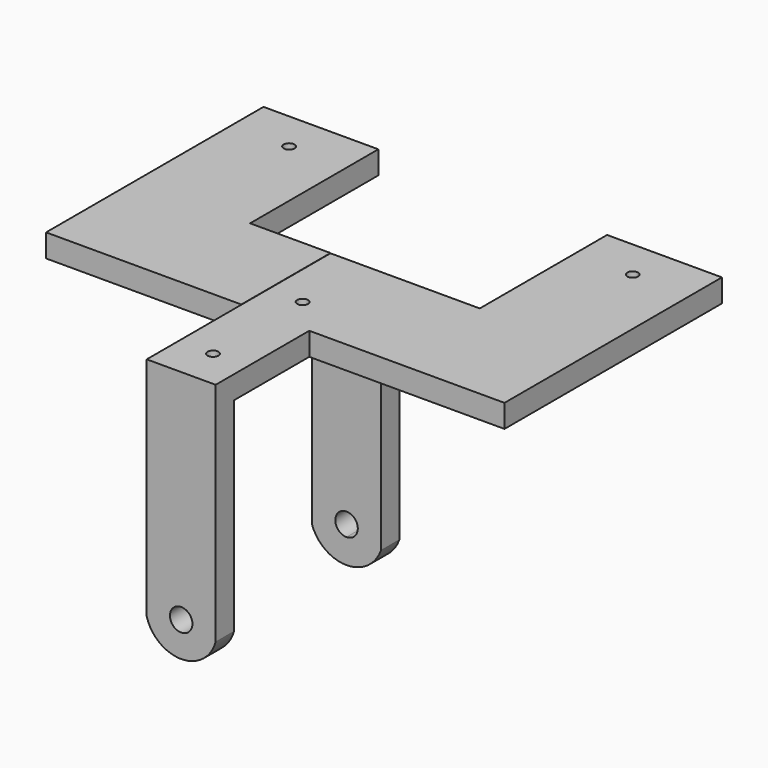
from build123d import *

# Parameters (mm, degrees)
F1_DEPTH  = 3.175
F2_DEPTH  = 3.175
F4_DEPTH  = 25.4
F5_DEPTH  = 25.4
F6_W      = 19.05
F6_H      = 63.5
F7_DEPTH  = 6.35
F9_DEPTH  = 6.35
F10_DEPTH = 2540
F11_R     = 1.5
F12_DEPTH = 25.4
F13_W     = 75.1403903484
F13_H     = 6.35
F14_DEPTH = 53.975
F15_R     = 1.5
F16_DEPTH = 25
F17_W     = 75.1403903484
F17_H     = 6.35
F18_DEPTH = 53.975
F19_R     = 1.5
F20_DEPTH = 25
F22_DEPTH = 22.225
F23_W     = 44.3243741632
F23_H     = 6.35
F24_DEPTH = 22.225


# Not quite as in the source:
# - a length typed as a fraction of an inch, garbled in the dataset ("3 / 203.2 mm" for 3/8 in), is restored


with BuildPart() as f1:
    # F0 (on Front) → F1 (new body)
    with BuildSketch(Plane.XZ):
        with BuildLine():
            Line((9.525, 25.206619263), (-9.525, 25.206619263))
            Line((-9.525, 25.206619263), (-9.525, -31.0143064708))
            ThreePointArc((-9.525, -31.0143064708), (0, -38.293380737), (9.525, -31.0143064708))
            Line((9.525, -31.0143064708), (9.525, 25.206619263))
        make_face()
    extrude(amount=F1_DEPTH)

    # F0 (on Front) → F2 (join)
    with BuildSketch(Plane.XZ):
        with BuildLine():
            Line((9.525, 25.206619263), (-9.525, 25.206619263))
            Line((-9.525, 25.206619263), (-9.525, -31.0143064708))
            ThreePointArc((-9.525, -31.0143064708), (0, -38.293380737), (9.525, -31.0143064708))
            Line((9.525, -31.0143064708), (9.525, 25.206619263))
        make_face()
    extrude(amount=-F2_DEPTH)

    # F3 (on Front) → F4 (cut)
    with BuildSketch(Plane.XZ):
        with BuildLine():
            ThreePointArc((0, -31.845793884), (2.2001627497, -30.9344566337), (3.1115, -28.734293884))
            ThreePointArc((3.1115, -28.734293884), (-2.2001627497, -26.5341311344), (0, -31.845793884))
        make_face()
    extrude(amount=-F4_DEPTH, mode=Mode.SUBTRACT)

    # F3 (on Front) → F5 (cut)
    with BuildSketch(Plane.XZ):
        with BuildLine():
            ThreePointArc((0, -31.845793884), (2.2001627497, -30.9344566337), (3.1115, -28.734293884))
            ThreePointArc((3.1115, -28.734293884), (-2.2001627497, -26.5341311344), (0, -31.845793884))
        make_face()
    extrude(amount=F5_DEPTH, mode=Mode.SUBTRACT)

    # F6 (on face) → F7 (join)
    with BuildSketch(Plane.XY.offset(25.206619263)):
        with Locations((0, 28.575)):
            Rectangle(F6_W, F6_H)
    extrude(amount=F7_DEPTH)

    # F11 (on face) → F12 (cut)
    with BuildSketch(Plane.XY.offset(31.556619263)):
        with Locations((0, 7.825)):
            Circle(F11_R)
        with Locations((0, 38.7934744358)):
            Circle(F11_R)
    extrude(amount=-F12_DEPTH, mode=Mode.SUBTRACT)



with BuildPart() as f9:
    # F8 (on face) → F9 (new body)
    with BuildSketch(Plane(origin=(0, 60.325, 0), x_dir=(-1, 0, 0), z_dir=(0, 1, 0))):
        with BuildLine():
            Line((-9.525, 31.556619263), (-9.525, -31.943380737))
            ThreePointArc((-9.525, -31.943380737), (0, -38.6772559995), (9.525, -31.943380737))
            Line((9.525, -31.943380737), (9.525, 31.556619263))
            Line((9.525, 31.556619263), (-9.525, 31.556619263))
        make_face()
    extrude(amount=-F9_DEPTH)

    # F3 (on Front) → F10 (cut)
    with BuildSketch(Plane.XZ):
        with BuildLine():
            ThreePointArc((0, -31.845793884), (2.2001627497, -30.9344566337), (3.1115, -28.734293884))
            ThreePointArc((3.1115, -28.734293884), (-2.2001627497, -26.5341311344), (0, -31.845793884))
        make_face()
    extrude(amount=-F10_DEPTH, mode=Mode.SUBTRACT)


with BuildPart() as f1_1:
    add(f1.part)

    add(f9.part)  # F14 merges F9
    # F13 (on face) → F14 (join)
    with BuildSketch(Plane.YZ.offset(9.525)):
        with Locations((66.7548048258, 28.381619263)):
            Rectangle(F13_W, F13_H)
    extrude(amount=F14_DEPTH)

    # F15 (on face) → F16 (cut)
    with BuildSketch(Plane.XY.offset(31.556619263)):
        with Locations((47.625, 93.325)):
            Circle(F15_R)
    extrude(amount=-F16_DEPTH, mode=Mode.SUBTRACT)

    # F17 (on face) → F18 (join)
    with BuildSketch(Plane(origin=(-9.525, 0, 0), x_dir=(0, -1, 0), z_dir=(-1, 0, 0))):
        with Locations((-67.0791789889, 28.4469667822)):
            Rectangle(F17_W, F17_H)
    extrude(amount=F18_DEPTH)

    # F19 (on face) → F20 (cut)
    with BuildSketch(Plane.XY.offset(31.6219667822)):
        with Locations((-47.625, 93.6493741632)):
            Circle(F19_R)
    extrude(amount=-F20_DEPTH, mode=Mode.SUBTRACT)

    # F21 (on face) → F22 (cut)
    with BuildSketch(Plane(origin=(9.525, 0, 0), x_dir=(0, -1, 0), z_dir=(-1, 0, 0))):
        Polygon((-104.325, 31.556619263), (-104.325, 25.206619263), (-61.1199513078, 25.206619263), (-60.325, 31.556619263), align=None)
    extrude(amount=-F22_DEPTH, mode=Mode.SUBTRACT)

    # F23 (on face) → F24 (cut)
    with BuildSketch(Plane.YZ.offset(-9.525)):
        with Locations((82.4871870816, 28.4469667822)):
            Rectangle(F23_W, F23_H)
    extrude(amount=-F24_DEPTH, mode=Mode.SUBTRACT)


solid = f1_1.part
